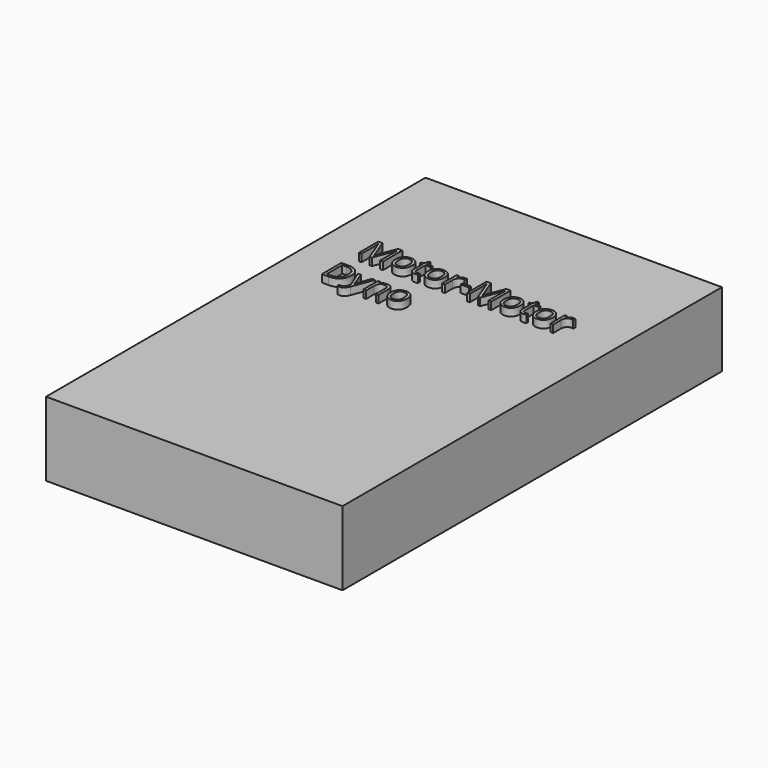
from build123d import *

# Parameters (mm, degrees)
F0_W         = 1000
F0_H         = 1600
F1_DEPTH     = 250
F2_TEXT_SIZE = 114.4404424349
F3_DEPTH     = 25.4


# Not quite as in the source:
# - Text() gives the source's letters only with a copy of the font that has no kerning and outlines rounded to 1/6400 em; it was checked with that copy


with BuildPart() as f1:
    # F0 (on Top) → F1 (new body)
    with BuildSketch(Plane.XY):
        Rectangle(F0_W, F0_H)
    extrude(amount=F1_DEPTH)

    # F2 (on face) → F3 (join)
    with BuildSketch(Plane.XY.offset(250)):
        with Locations((-350, 317.6028814469)):
            Text('Motor-Motor', F2_TEXT_SIZE, font='Open Sans', text_align=(TextAlign.LEFT, TextAlign.BOTTOM))
        with Locations((-350, 161.9638797354)):
            Text('Dyno', F2_TEXT_SIZE, font='Open Sans', text_align=(TextAlign.LEFT, TextAlign.BOTTOM))
    extrude(amount=F3_DEPTH)


solid = f1.part
